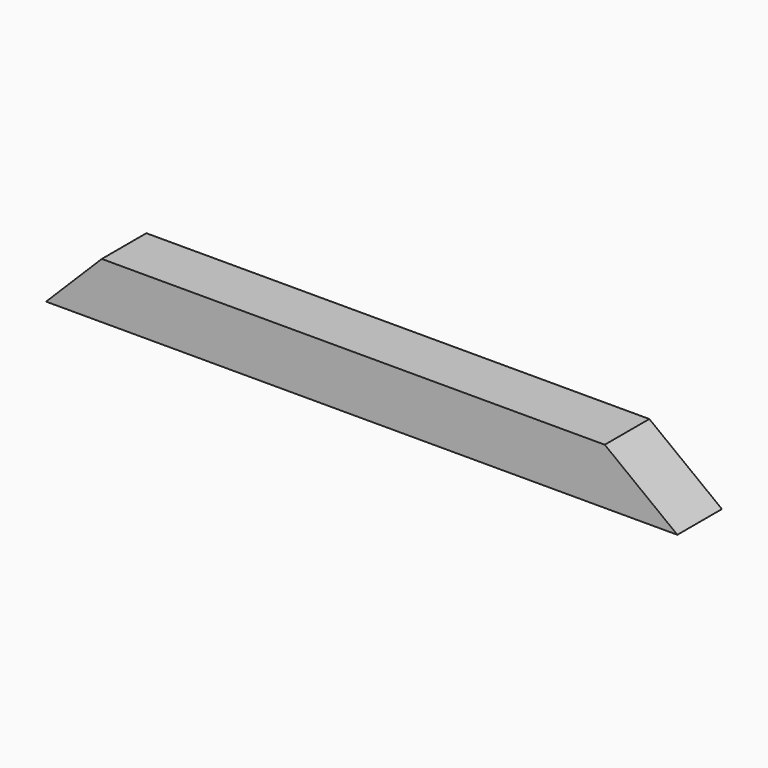
from build123d import *

# Parameters (mm, degrees)
F1_DEPTH = 19.05
F2_SIZE  = 38.09999


# Not quite as in the source:
# - a fillet or chamfer is up to 0.001 mm smaller than in the source, because OpenCascade refuses the exact size


with BuildPart() as f1:
    # F0 (on Front) → F1 (new body, symmetric)
    with BuildSketch(Plane.XZ):
        Polygon((-215.9, 19.05), (-215.9, -19.05), (215.9, -19.05), (166.2471132948, 19.05), align=None)
    extrude(amount=F1_DEPTH, both=True)

    # F2 (size 38.1 in the source; OpenCascade refuses exactly that, so slightly less here)
    f2_edges = [f1.edges().sort_by_distance(p)[0] for p in [
        (-215.9, 0, 19.05),
    ]]
    chamfer(f2_edges, length=F2_SIZE)


solid = f1.part
